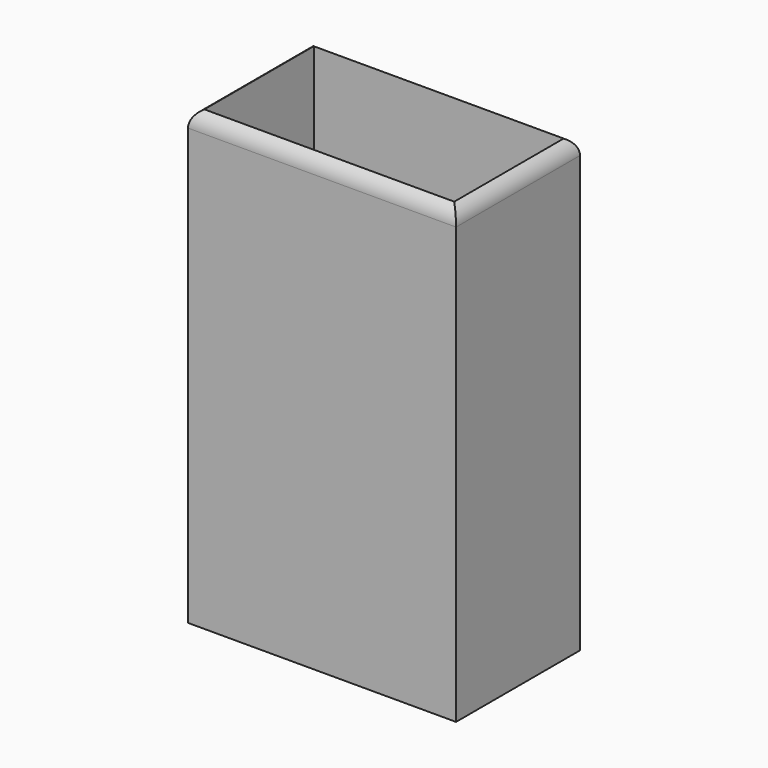
from build123d import *

# Parameters (mm, degrees)
F0_W        = 75.0152692199
F0_H        = 43.3505326509
F1_DEPTH    = 127
F2_T        = -2.54
F3_T1_DEPTH = 100.4152692199
F3_T3_DEPTH = 68.7505326509


# Not quite as in the source:
# - a fillet or chamfer that OpenCascade refuses, or shapes differently, is made with other operations: its cross-section is extruded or revolved along the edge and cut away or added


with BuildPart() as f1:
    # F0 (on Top) → F1 (new body)
    with BuildSketch(Plane.XY):
        with Locations((1.8848069012, 0.6596818566)):
            Rectangle(F0_W, F0_H)
    extrude(amount=F1_DEPTH)

    # F2
    f2_openings = [f1.faces().sort_by_distance(p)[0] for p in [
        (1.884807, 0.659682, 127),
    ]]
    offset(amount=F2_T, openings=f2_openings)

    # F3: fillet of radius 5.08 on 4 edges, made by hand

    # F3_s2 → F3_t1 (cut)
    with BuildSketch(Plane.YZ.offset(-48.3228277087)):
        with BuildLine():
            ThreePointArc((22.3349481821, 121.92), (20.8470506305, 125.5121024484), (17.2549481821, 127))
            Line((17.2549481821, 127), (22.3349481821, 127))
            Line((22.3349481821, 127), (22.3349481821, 121.92))
        make_face()
        with BuildLine():
            ThreePointArc((-21.0155844688, 121.92), (-19.5276869173, 125.5121024484), (-15.9355844688, 127))
            Line((-15.9355844688, 127), (-21.0155844688, 127))
            Line((-21.0155844688, 127), (-21.0155844688, 121.92))
        make_face()
    extrude(amount=F3_T1_DEPTH, mode=Mode.SUBTRACT)

    # F3_s4 → F3_t3 (cut)
    with BuildSketch(Plane.XZ.offset(-35.0349481821)):
        with BuildLine():
            ThreePointArc((-35.6228277087, 121.92), (-34.1349301571, 125.5121024484), (-30.5428277087, 127))
            Line((-30.5428277087, 127), (-35.6228277087, 127))
            Line((-35.6228277087, 127), (-35.6228277087, 121.92))
        make_face()
        with BuildLine():
            ThreePointArc((39.3924415112, 121.92), (37.9045439596, 125.5121024484), (34.3124415112, 127))
            Line((34.3124415112, 127), (39.3924415112, 127))
            Line((39.3924415112, 127), (39.3924415112, 121.92))
        make_face()
    extrude(amount=F3_T3_DEPTH, mode=Mode.SUBTRACT)


solid = f1.part
